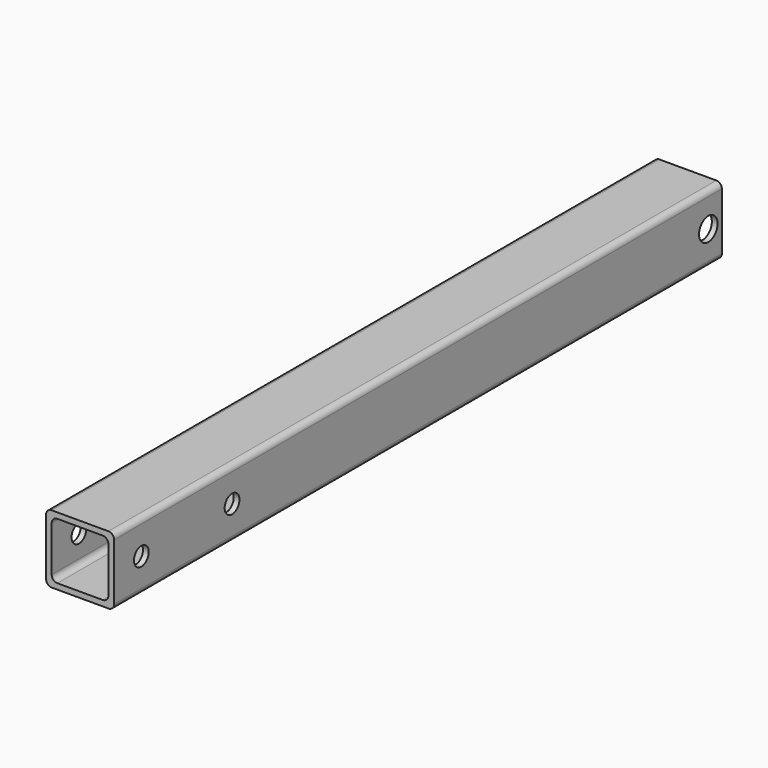
from build123d import *

# Parameters (mm, degrees)
F0_W     = 19.05
F0_H     = 19.05
F0_W_2   = 15.875
F0_H_2   = 15.875
F1_DEPTH = 107.95
F2_R     = 1.5875
F3_R     = 1.5875
F4_R     = 3.2385
F4_R_2   = 2.5796875
F5_DEPTH = 19.05
F6_DEPTH = 3.175


# Not quite as in the source:
# - a length typed as a fraction of an inch, garbled in the dataset ("3 / 203.2 mm" for 3/8 in), is restored


with BuildPart() as f1:
    # F0 (on Front) → F1 (new body, symmetric)
    with BuildSketch(Plane.XZ):
        Rectangle(F0_W, F0_H)
        with Locations((-0.0127, 0)):
            Rectangle(F0_W_2, F0_H_2, mode=Mode.SUBTRACT)
    extrude(amount=F1_DEPTH, both=True)

    # F2
    f2_edges = [f1.edges().sort_by_distance(p)[0] for p in [
        (-9.525, 0, 9.525),
        (-9.525, 0, -9.525),
        (9.525, 0, -9.525),
        (9.525, 0, 9.525),
    ]]
    fillet(f2_edges, radius=F2_R)

    # F3
    f3_edges = [f1.edges().sort_by_distance(p)[0] for p in [
        (-7.9502, 0, 7.9375),
        (-7.9502, 0, -7.9375),
        (7.9248, 0, 7.9375),
        (7.9248, 0, -7.9375),
    ]]
    fillet(f3_edges, radius=F3_R)

    # F4 (on face) → F5 (cut)
    with BuildSketch(Plane(origin=(-9.525, 0, 0), x_dir=(0, -1, 0), z_dir=(-1, 0, 0))):
        with Locations((-103.1875, 0)):
            Circle(F4_R)
        with Locations((63.5, 0)):
            Circle(F4_R_2)
        with Locations((95.25, 0)):
            Circle(F4_R_2)
    extrude(amount=-F5_DEPTH, mode=Mode.SUBTRACT)

    # F6 (cut): a face of the model
    f6_faces = [f1.faces().sort_by_distance(p)[0] for p in [
        (-8.2196076836, -107.95, 0),
    ]]
    extrude(f6_faces, amount=-F6_DEPTH, mode=Mode.SUBTRACT)


solid = f1.part
